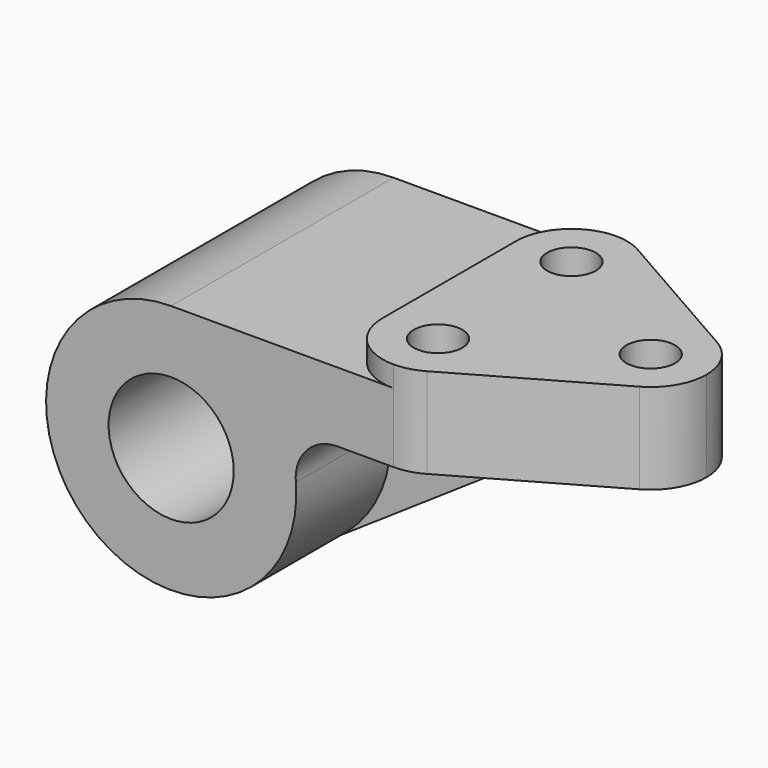
from build123d import *

# Parameters (mm, degrees)
F0_R     = 14.2875
F1_DEPTH = 31.75
F2_DEPTH = 4.7625
F4_DEPTH = 25.4
F5_DEPTH = 25.4
F6_DEPTH = 4.7752
F3_R     = 5.5626
F7_DEPTH = 25.4


with BuildPart() as f1:
    # F0 (on Front) → F1 (new body, symmetric)
    with BuildSketch(Plane.XZ):
        with BuildLine():
            Line((38.1, 28.575), (0, 28.575))
            ThreePointArc((0, 28.575), (-27.3235693319, -8.3638020041), (15.9950252975, -23.6788891364))
            ThreePointArc((15.9950252975, -23.6788891364), (25.7719232537, -12.3425522809), (28.4756083945, 2.38125))
            ThreePointArc((28.4756083945, 2.38125), (30.9572676717, 9.6234554837), (37.9674778593, 12.7))
            Line((37.9674778593, 12.7), (69.85, 12.7))
            Line((69.85, 12.7), (96.8502, 12.7))
            Line((96.8502, 12.7), (96.8502, 33.3502))
            Line((96.8502, 33.3502), (38.1, 33.3502))
            Line((38.1, 33.3502), (38.1, 28.575))
        make_face()
        Circle(F0_R, mode=Mode.SUBTRACT)
    extrude(amount=F1_DEPTH, both=True)

    # F0 (on Front) → F2 (join, symmetric)
    with BuildSketch(Plane.XZ):
        with BuildLine():
            ThreePointArc((28.4756083945, 2.38125), (25.7719232537, -12.3425522809), (15.9950252975, -23.6788891364))
            Line((15.9950252975, -23.6788891364), (69.85, 12.7))
            Line((69.85, 12.7), (37.9674778593, 12.7))
            ThreePointArc((37.9674778593, 12.7), (30.9572676717, 9.6234554837), (28.4756083945, 2.38125))
        make_face()
    extrude(amount=F2_DEPTH, both=True)

    # F3 (on face) → F4 (cut)
    with BuildSketch(Plane.XY.offset(33.3502)):
        with BuildLine():
            ThreePointArc((50.8, 31.75), (54.0586759125, 31.3248128824), (57.0991554441, 30.0777214642))
            Line((57.0991554441, 30.0777214642), (90.4493554441, 11.0277214642))
            ThreePointArc((90.4493554441, 11.0277214642), (95.1340352623, 6.3753715915), (96.8502, 0))
            Line((96.8502, 0), (96.8502, 31.75))
            Line((96.8502, 31.75), (50.8, 31.75))
        make_face()
    extrude(amount=-F4_DEPTH, mode=Mode.SUBTRACT)

    # F3 (on face) → F5 (cut)
    with BuildSketch(Plane.XY.offset(33.3502)):
        with BuildLine():
            Line((96.8502, -31.75), (96.8502, 0))
            ThreePointArc((96.8502, 0), (95.1340352623, -6.3753715915), (90.4493554441, -11.0277214642))
            Line((90.4493554441, -11.0277214642), (57.0991554441, -30.0777214642))
            ThreePointArc((57.0991554441, -30.0777214642), (54.0586759125, -31.3248128824), (50.8, -31.75))
            Line((50.8, -31.75), (96.8502, -31.75))
        make_face()
    extrude(amount=-F5_DEPTH, mode=Mode.SUBTRACT)

    # F3 (on face) → F6 (cut)
    with BuildSketch(Plane.XY.offset(33.3502)):
        with BuildLine():
            ThreePointArc((50.8, -31.75), (41.8197438789, -28.0302561211), (38.1, -19.05))
            Line((38.1, -19.05), (38.1, -31.75))
            Line((38.1, -31.75), (50.8, -31.75))
        make_face()
        with BuildLine():
            ThreePointArc((38.1, 19.05), (41.8197438789, 28.0302561211), (50.8, 31.75))
            Line((50.8, 31.75), (38.1, 31.75))
            Line((38.1, 31.75), (38.1, 19.05))
        make_face()
    extrude(amount=-F6_DEPTH, mode=Mode.SUBTRACT)

    # F3 (on face) → F7 (cut)
    with BuildSketch(Plane.XY.offset(33.3502)):
        with Locations((84.1502, 0)):
            Circle(F3_R)
        with Locations((50.8, 19.05)):
            Circle(F3_R)
        with Locations((50.8, -19.05)):
            Circle(F3_R)
    extrude(amount=-F7_DEPTH, mode=Mode.SUBTRACT)


solid = f1.part
